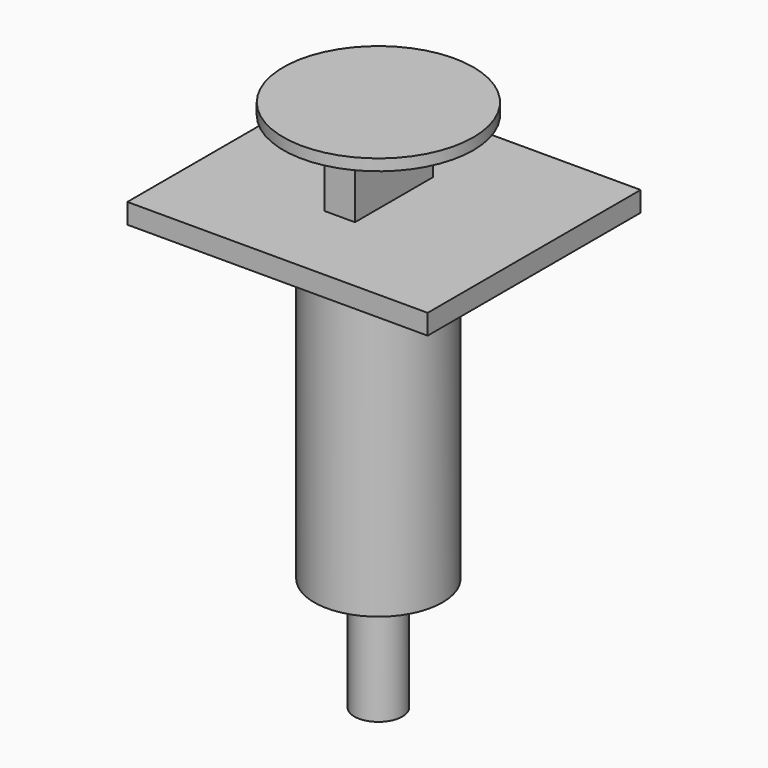
from build123d import *

# Parameters (mm, degrees)
F0_R      = 8.33
F0_R_2    = 7.2338998847
F1_DEPTH  = 41.3
F0_R_3    = 3.120788822
F3_DEPTH  = 1.778
F4_DEPTH  = 14.732
F6_DEPTH  = 17.272
F7_W      = 3.9808914298
F7_H      = 9.0002007782
F8_DEPTH  = 6.35
F11_R     = 12.3283850527
F11_W     = 3.9808914298
F11_H     = 12.7
F12_DEPTH = 1.4732


# Not quite as in the source:
# - the program builds the solid bodies; features that only make, move or delete a surface that nothing else refers to are left out


with BuildPart() as f1:
    # F0 (on Top) → F1 (new body)
    with BuildSketch(Plane.XY):
        Circle(F0_R)
        Circle(F0_R_2, mode=Mode.SUBTRACT)
    extrude(amount=F1_DEPTH)

    # F0 (on Top) → F3 (join)
    with BuildSketch(Plane.XY):
        Circle(F0_R_2)
        Circle(F0_R_3, mode=Mode.SUBTRACT)
    extrude(amount=F3_DEPTH)


with BuildPart() as f4:
    # F0 (on Top) → F4 (new body)
    with BuildSketch(Plane.XY):
        Circle(F0_R_3)
    extrude(amount=-F4_DEPTH)


with BuildPart() as f6:
    # F5 (on Front) → F6 (new body, symmetric)
    with BuildSketch(Plane.XZ):
        Polygon((-18.754336983, 41.362978518), (0, 41.362978518), (20.2109832317, 41.362978518), (20.2109832317, 43.9725443721), (-18.754336983, 43.9725443721), align=None)
    extrude(amount=F6_DEPTH, both=True)


with BuildPart() as f8:
    # F7 (on Front) → F8 (new body, symmetric)
    with BuildSketch(Plane.XZ):
        with Locations((0.0484315096, 48.4631862491)):
            Rectangle(F7_W, F7_H)
    extrude(amount=F8_DEPTH, both=True)

    # F11 (on face) → F12 (join)
    with BuildSketch(Plane.XY.offset(52.9632866383)):
        Circle(F11_R)
        with Locations((0.0484315096, 0)):
            Rectangle(F11_W, F11_H, mode=Mode.SUBTRACT)
        Circle(F11_R)
    extrude(amount=F12_DEPTH)


solid = Compound([f1.part, f4.part, f6.part, f8.part])
